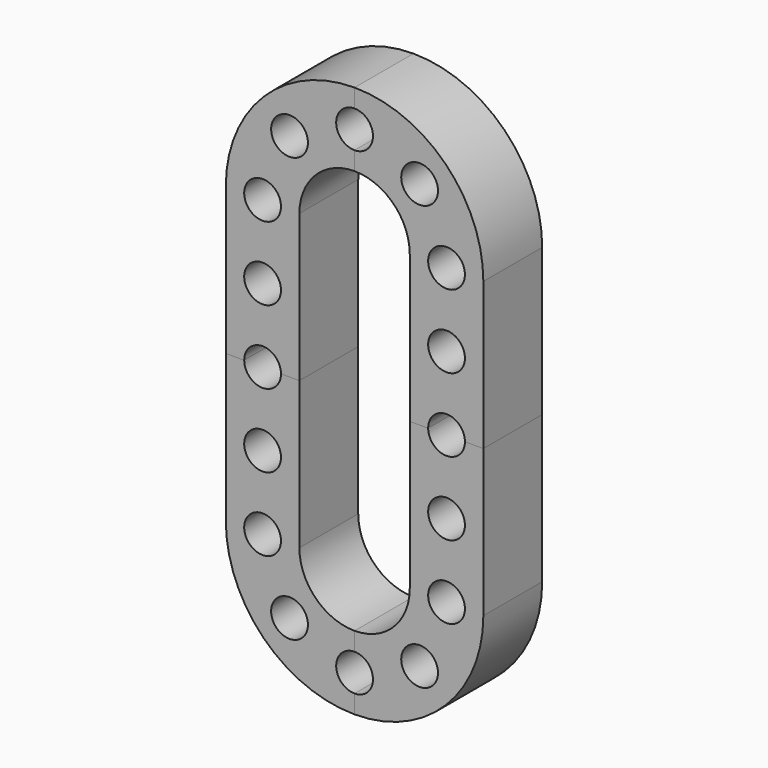
from build123d import *
from build123d import SkipClean  # not in build123d's __all__

# Parameters (mm, degrees)
F0_R     = 5
F1_DEPTH = 20


with BuildPart() as f1:
    # F0 (on Front) → F1 (new body)
    with BuildSketch(Plane.XZ):
        with BuildLine():
            ThreePointArc((-15, 40), (-10.6066017178, 50.6066017178), (0, 55))
            Line((0, 55), (0, 60))
            ThreePointArc((0, 60), (-5, 65), (0, 70))
            Line((0, 70), (0, 75))
            ThreePointArc((0, 75), (-24.7487373415, 64.7487373415), (-35, 40))
            Line((-35, 40), (-35, 0))
            Line((-35, 0), (-30, 0))
            ThreePointArc((-30, 0), (-25, 5), (-20, 0))
            Line((-20, 0), (-15, 0))
            Line((-15, 0), (-15, 40))
        make_face()
        with Locations((-25, 20)):
            Circle(F0_R, mode=Mode.SUBTRACT)
        with Locations((-25, 40)):
            Circle(F0_R, mode=Mode.SUBTRACT)
        with Locations((-17.6776695297, 57.6776695297)):
            Circle(F0_R, mode=Mode.SUBTRACT)
    extrude(amount=F1_DEPTH)

    # F2: F1 across plane


with BuildPart() as f1_1:
    add(f1.part, clean=False)
    with SkipClean():  # cleaning this boolean's faces spoils the solid; the shape is the same uncleaned
        add(f1.part.mirror(Plane.XY), clean=False)

    # F3: F1 across plane


with BuildPart() as f1_2:
    add(f1_1.part, clean=False)
    with SkipClean():  # cleaning this boolean's faces spoils the solid; the shape is the same uncleaned
        add(f1_1.part.mirror(Plane.YZ), clean=False)


solid = f1_2.part
